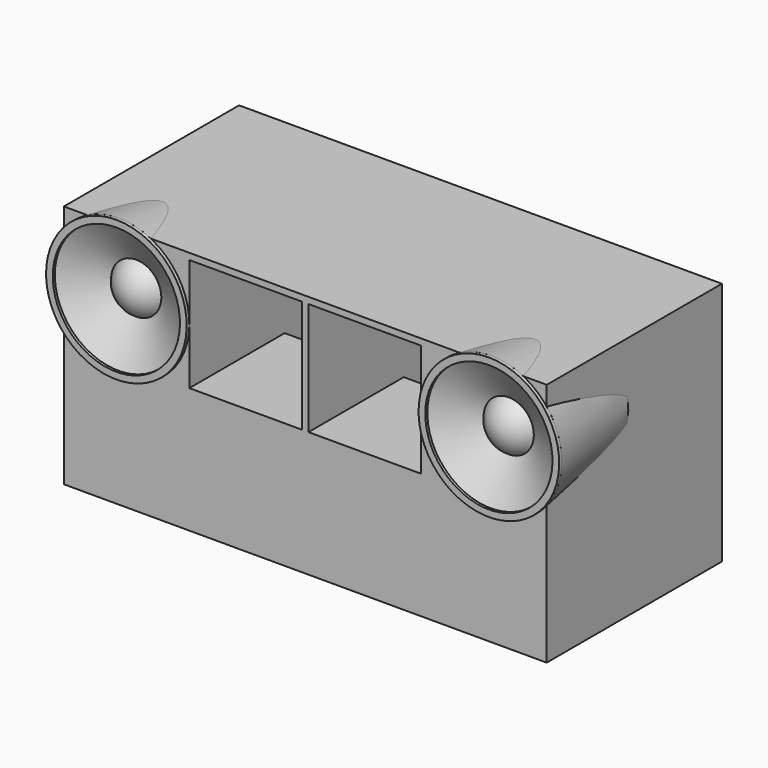
from build123d import *

# Parameters (mm, degrees)
F3_W      = 730.5324633441
F3_H      = 654.0714285714
F4_DEPTH  = 336.766231672
F6_DEPTH  = 730.5324633441
F7_W      = 730.5324633441
F7_H      = 654.0714285714
F7_W_2    = 336.766231672
F7_H_2    = 279.3051968994
F8_DEPTH  = 19
F9_W      = 730.5324633441
F9_H      = 654.0714285714
F9_W_2    = 336.766231672
F9_H_2    = 616.0714285714
F10_DEPTH = 336.766231672
F12_DEPTH = 730.5324633441
F13_W     = 730.5324633441
F13_H     = 654.0714285714
F14_DEPTH = 19
F15_W     = 730.5324633441
F15_H     = 654.0714285714
F16_DEPTH = 19
F17_W     = 336.766231672
F17_H     = 336.766231672
F18_DEPTH = 25
F22_R     = 190
F23_DEPTH = 19


with BuildPart() as f4:
    # F3 (on Top) → F4 (new body)
    with BuildSketch(Plane.XY):
        with Locations((-355.766231672, 327.0357142857)):
            Rectangle(F3_W, F3_H)
        Polygon((-392.1362893571, 19), (-702.0324633441, 19), (-702.0324633441, 328.896173987), align=None, mode=Mode.SUBTRACT)
        Polygon((-702.0324633441, 355.766231672), (-702.0324633441, 635.0714285714), (-365.266231672, 635.0714285714), (-365.266231672, 355.766231672), (-346.266231672, 355.766231672), (-346.266231672, 635.0714285714), (-9.5, 635.0714285714), (-9.5, 355.766231672), (-346.266231672, 19), (-365.266231672, 19), align=None, mode=Mode.SUBTRACT)
        Polygon((-9.5, 19), (-319.396173987, 19), (-9.5, 328.896173987), align=None, mode=Mode.SUBTRACT)
    extrude(amount=F4_DEPTH)

    # F5 (on face) → F6 (join, through all)
    with BuildSketch(Plane(origin=(-721.0324633441, 0, 0), x_dir=(0, -1, 0), z_dir=(-1, 0, 0))):
        Polygon((-298.3051968994, 0), (-635.0714285714, 336.766231672), (-635.0714285714, 309.896173987), (-325.1752545845, 0), align=None)
    extrude(amount=-F6_DEPTH)

    # F7 (on face) → F8 (join)
    with BuildSketch(Plane.XY.offset(336.766231672)):
        with Locations((-355.766231672, 327.0357142857)):
            Rectangle(F7_W, F7_H)
        with Locations((-533.6493475081, 495.4188301217)):
            Rectangle(F7_W_2, F7_H_2, mode=Mode.SUBTRACT)
        with Locations((-177.883115836, 495.4188301217)):
            Rectangle(F7_W_2, F7_H_2, mode=Mode.SUBTRACT)
    extrude(amount=F8_DEPTH)

    # F9 (on face) → F10 (join)
    with BuildSketch(Plane.XY.offset(355.766231672)):
        with Locations((-355.766231672, 327.0357142857)):
            Rectangle(F9_W, F9_H)
        with Locations((-533.6493475081, 327.0357142857)):
            Rectangle(F9_W_2, F9_H_2, mode=Mode.SUBTRACT)
        with Locations((-177.883115836, 327.0357142857)):
            Rectangle(F9_W_2, F9_H_2, mode=Mode.SUBTRACT)
    extrude(amount=F10_DEPTH)

    # F11 (on face) → F12 (join, through all)
    with BuildSketch(Plane(origin=(-721.0324633441, 0, 0), x_dir=(0, -1, 0), z_dir=(-1, 0, 0))):
        Polygon((-296.7492855239, 692.5324633441), (-323.619343209, 692.5324633441), (-635.0714285714, 381.0803779817), (-635.0714285714, 354.2103202966), align=None)
    extrude(amount=-F12_DEPTH)

    # F13 (on face) → F14 (join)
    with BuildSketch(Plane.XY.offset(692.5324633441)):
        with Locations((-355.766231672, 327.0357142857)):
            Rectangle(F13_W, F13_H)
    extrude(amount=F14_DEPTH)

    # F15 (on face) → F16 (join)
    with BuildSketch(Plane(origin=(0, 0, 0), x_dir=(1, 0, 0), z_dir=(0, 0, -1))):
        with Locations((-355.766231672, -327.0357142857)):
            Rectangle(F15_W, F15_H)
    extrude(amount=F16_DEPTH)

    # F17 (on face) → F18 (cut)
    with BuildSketch(Plane.XZ):
        with Locations((-177.883115836, 524.1493475081)):
            Rectangle(F17_W, F17_H)
    extrude(amount=-F18_DEPTH, mode=Mode.SUBTRACT)

    # F20 (on offset) → F21 (revolve)
    with BuildSketch(Plane.YZ.offset(-556.266231672)):
        Polygon((300, 524.1493475081), (0, 524.1493475081), (0, 314.1493475081), (300, 355.766231672), align=None)
    revolve(axis=Axis((-556.266231672, 150, 524.1493475081), (0, 1, 0)))

    # F22 (on face) → F23 (cut)
    with BuildSketch(Plane.XZ):
        with Locations((-556.266231672, 524.1493475081)):
            Circle(F22_R)
    extrude(amount=-F23_DEPTH, mode=Mode.SUBTRACT)

    # F24 (on offset) → F25 (revolve, cut)
    with BuildSketch(Plane.YZ.offset(-556.266231672)):
        Polygon((0, 714.1493475081), (0, 524.1493475081), (300, 524.1493475081), (300, 692.5324633441), align=None)
    revolve(axis=Axis((-556.266231672, 150, 524.1493475081), (0, 1, 0)), mode=Mode.SUBTRACT)

    # F26: F4 across plane


with BuildPart() as f4_1:
    add(f4.part)
    add(f4.part.mirror(Plane.YZ))


with BuildPart() as f28:
    # F27 (on offset) → F28 (revolve)
    with BuildSketch(Plane.YZ.offset(-556.266231672)):
        with BuildLine():
            Line((0, 734.1493475081), (-10, 734.1493475081))
            Line((-10, 734.1493475081), (-10, 714.1493475081))
            Line((-10, 714.1493475081), (-2.3094010768, 714.1493475081))
            Line((-2.3094010768, 714.1493475081), (64.08587988, 599.1493475081))
            ThreePointArc((64.08587988, 599.1493475081), (32.3871500693, 567.4506176973), (20.7846096908, 524.1493475081))
            Line((20.7846096908, 524.1493475081), (109.696551146, 524.1493475081))
            Line((109.696551146, 524.1493475081), (0, 714.1493475081))
            Line((0, 714.1493475081), (0, 734.1493475081))
        make_face()
    revolve(axis=Axis((-556.266231672, 103.9801740821, 524.1493475081), (0, 1, 0)))


with BuildPart() as f29_1:
    # F29: instance of F28
    add(f28.part.mirror(Plane.YZ))


solid = Compound([f4_1.part, f28.part, f29_1.part])
